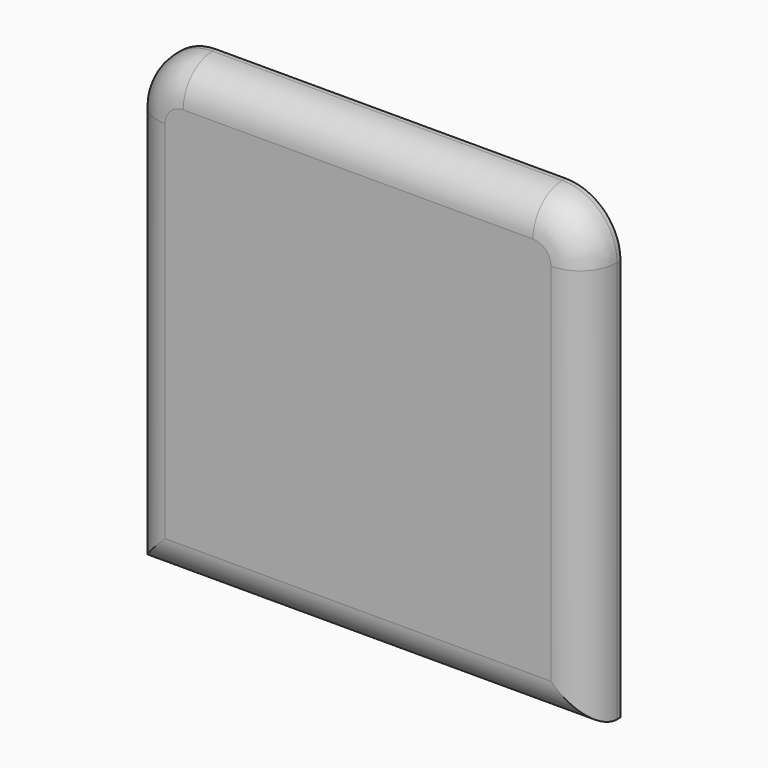
from build123d import *

# Parameters (mm, degrees)
F0_W        = 85.2935686707
F0_H        = 84.8211869597
F0_R        = 1.905
F0_R_2      = 0.8509
F1_DEPTH    = 7.62
F2_R        = 6.8125926862
F3_T1_DEPTH = 33.02
F3_T4_ANGLE = 90
F3_T6_ANGLE = 90


# Not quite as in the source:
# - a fillet or chamfer that OpenCascade refuses, or shapes differently, is made with other operations: its cross-section is extruded or revolved along the edge and cut away or added


with BuildPart() as f1:
    # F0 (on Front) → F1 (new body)
    with BuildSketch(Plane.XZ):
        Rectangle(F0_W, F0_H)
        Polygon((0, 38.1), (38.1, 38.1), (38.1, -38.1), (0, -38.1), (-38.1, -38.1), (-38.1, 38.1), align=None, mode=Mode.SUBTRACT)
        Polygon((25.4, 25.4), (0, 25.4), (-25.4, 25.4), (-25.4, -25.4), (0, -25.4), (25.4, -25.4), align=None)
        with Locations((-18.288, -12.446)):
            Circle(F0_R, mode=Mode.SUBTRACT)
        with Locations((19.812, -12.446)):
            Circle(F0_R, mode=Mode.SUBTRACT)
        with Locations((-18.288, 12.954)):
            Circle(F0_R, mode=Mode.SUBTRACT)
        with Locations((19.812, 12.954)):
            Circle(F0_R, mode=Mode.SUBTRACT)
        Polygon((0, 25.4), (0, 38.1), (-38.1, 38.1), (-38.1, -38.1), (0, -38.1), (0, -25.4), (-25.4, -25.4), (-25.4, 25.4), align=None)
        Polygon((38.1, -38.1), (38.1, 38.1), (0, 38.1), (0, 25.4), (25.4, 25.4), (25.4, -25.4), (0, -25.4), (0, -38.1), align=None)
        with Locations((-18.288, -12.446)):
            Circle(F0_R)
        with Locations((-18.288, -12.446)):
            Circle(F0_R_2, mode=Mode.SUBTRACT)
        with Locations((-18.288, 12.954)):
            Circle(F0_R)
        with Locations((-18.288, 12.954)):
            Circle(F0_R_2, mode=Mode.SUBTRACT)
        with Locations((19.812, 12.954)):
            Circle(F0_R)
        with Locations((19.812, 12.954)):
            Circle(F0_R_2, mode=Mode.SUBTRACT)
        with Locations((19.812, -12.446)):
            Circle(F0_R)
        with Locations((19.812, -12.446)):
            Circle(F0_R_2, mode=Mode.SUBTRACT)
        with Locations((-18.288, 12.954)):
            Circle(F0_R_2)
        with Locations((-18.288, -12.446)):
            Circle(F0_R_2)
        with Locations((19.812, 12.954)):
            Circle(F0_R_2)
        with Locations((19.812, -12.446)):
            Circle(F0_R_2)
    extrude(amount=F1_DEPTH)

    # F2
    f2_edges = [f1.edges().sort_by_distance(p)[0] for p in [
        (0, -7.62, -42.410593),
        (-42.646784, -7.62, 0),
        (0, -7.62, 42.410593),
        (42.646784, -7.62, 0),
    ]]
    fillet(f2_edges, radius=F2_R)

    # F3: fillet of radius 10.16 on 2 edges, made by hand

    # F3_s2 → F3_t1 (cut)
    with BuildSketch(Plane.XZ.offset(-25.4)):
        with BuildLine():
            ThreePointArc((42.6467843354, 32.2505934799), (39.6709892322, 39.4347983767), (32.4867843354, 42.4105934799))
            Line((32.4867843354, 42.4105934799), (42.6467843354, 42.4105934799))
            Line((42.6467843354, 42.4105934799), (42.6467843354, 32.2505934799))
        make_face()
        with BuildLine():
            ThreePointArc((-32.4867843354, 42.4105934799), (-39.6709892322, 39.4347983767), (-42.6467843354, 32.2505934799))
            Line((-42.6467843354, 32.2505934799), (-42.6467843354, 42.4105934799))
            Line((-42.6467843354, 42.4105934799), (-32.4867843354, 42.4105934799))
        make_face()
    extrude(amount=F3_T1_DEPTH, mode=Mode.SUBTRACT)

    # F3_s3 → F3_t4 (revolve, cut)
    with BuildSketch(Plane.YZ.offset(-32.4867843354)):
        with BuildLine():
            ThreePointArc((-7.62, 35.5980007937), (-5.6246377997, 40.4152312796), (-0.8074073138, 42.4105934799))
            Line((-0.8074073138, 42.4105934799), (-7.62, 42.4105934799))
            Line((-7.62, 42.4105934799), (-7.62, 35.5980007937))
        make_face()
    revolve(axis=Axis((-32.4867843354, -7.62, 32.2505934799), (0, -1, 0)), revolution_arc=F3_T4_ANGLE, mode=Mode.SUBTRACT)

    # F3_s5 → F3_t6 (revolve, cut)
    with BuildSketch(Plane.XY.offset(32.2505934799)):
        with BuildLine():
            ThreePointArc((35.8341916492, -7.62), (40.6514221351, -5.6246377997), (42.6467843354, -0.8074073138))
            Line((42.6467843354, -0.8074073138), (42.6467843354, -7.62))
            Line((42.6467843354, -7.62), (35.8341916492, -7.62))
        make_face()
    revolve(axis=Axis((32.4867843354, -7.62, 32.2505934799), (0, -1, 0)), revolution_arc=F3_T6_ANGLE, mode=Mode.SUBTRACT)


solid = f1.part
